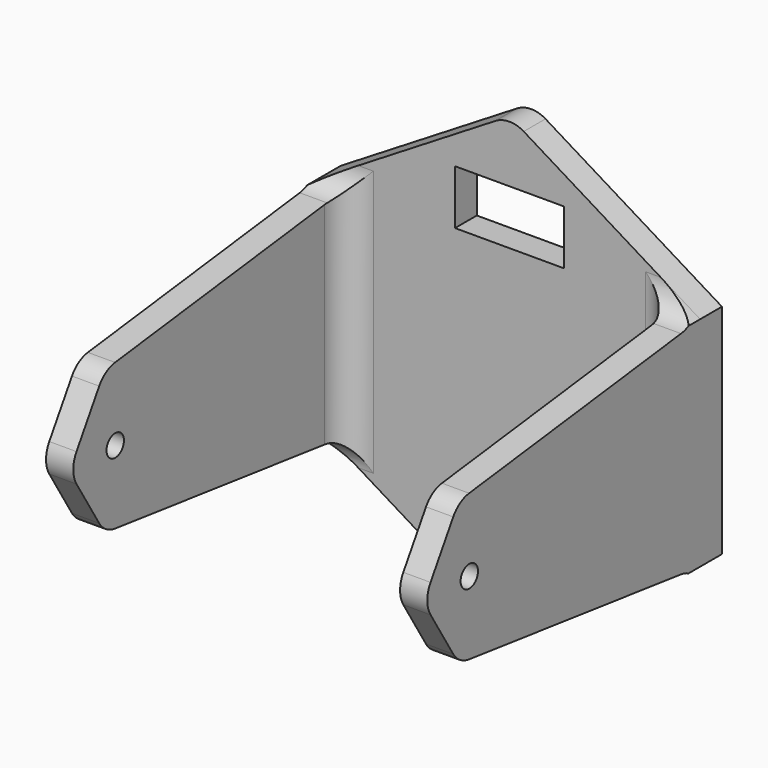
from build123d import *

# Parameters (mm, degrees)
F0_W         = 5
F0_H         = 40
F1_DEPTH     = 70
F3_DEPTH     = 5
F4_R         = 2
F5_DEPTH     = 97.2
F7_DEPTH     = 83.6
F8_T4_DEPTH  = 65
F8_T10_DEPTH = 65
F8_T16_DEPTH = 5
F8_T21_DEPTH = 5
F8_T26_DEPTH = 5
F8_T31_DEPTH = 5
F8_T37_DEPTH = 16.0458347789
F8_T42_DEPTH = 65
F8_T50_DEPTH = 16.0458347789
F8_T55_DEPTH = 65
F8_T63_DEPTH = 16.0458347789
F8_T68_DEPTH = 65
F8_T76_DEPTH = 65
F8_T81_DEPTH = 16.0458347789
F8_T85_DEPTH = 20.294112478
F9_W         = 20
F9_H         = 10
F10_DEPTH    = 25


# Not quite as in the source:
# - a fillet or chamfer that OpenCascade refuses, or shapes differently, is made with other operations: its cross-section is extruded or revolved along the edge and cut away or added


with BuildPart() as f1:
    # F0 (on Front) → F1 (new body)
    with BuildSketch(Plane.XZ):
        with Locations((-32.5, 0)):
            Rectangle(F0_W, F0_H)
    extrude(amount=F1_DEPTH)



with BuildPart() as f1b:
    # F0 (on Front) → F1, piece 2 (new body)
    with BuildSketch(Plane.XZ):
        with Locations((32.5, 0)):
            Rectangle(F0_W, F0_H)
    extrude(amount=F1_DEPTH)


with BuildPart() as f1_1:
    add(f1.part)

    add(f1b.part)  # F3 merges F1b
    # F2 (on face) → F3 (join)
    with BuildSketch(Plane(origin=(0, 0, 0), x_dir=(-1, 0, 0), z_dir=(0, 1, 0))):
        Polygon((-35, -20), (0, -41.4117574692), (35, -20), (35, 20), (0, 41.4117574692), (-35, 20), align=None)
    extrude(amount=F3_DEPTH)

    # F4 (on face) → F5 (cut)
    with BuildSketch(Plane(origin=(-35, 0, 0), x_dir=(0, -1, 0), z_dir=(-1, 0, 0))):
        with Locations((52.9787652194, 0)):
            Circle(F4_R)
    extrude(amount=-F5_DEPTH, mode=Mode.SUBTRACT)

    # F6 (on face) → F7 (cut)
    with BuildSketch(Plane(origin=(-35, 0, 0), x_dir=(0, -1, 0), z_dir=(-1, 0, 0))):
        with BuildLine():
            Line((98.4306931496, 40.8057309687), (0, 20))
            Line((0, 20), (53.01884554, 13.4261534673))
            ThreePointArc((53.01884554, 13.4261534673), (55.107028482, 12.6702755654), (56.6618948527, 11.084636902))
            Line((56.6618948527, 11.084636902), (61.8706015463, 2.6204867239))
            ThreePointArc((61.8706015463, 2.6204867239), (62.6123097139, 0), (61.8706015463, -2.6204867239))
            Line((61.8706015463, -2.6204867239), (56.6618948527, -11.084636902))
            ThreePointArc((56.6618948527, -11.084636902), (55.107028482, -12.6702755654), (53.01884554, -13.4261534673))
            Line((53.01884554, -13.4261534673), (0, -20))
            Line((0, -20), (98.4306931496, -42.0177839696))
            Line((98.4306931496, -42.0177839696), (98.4306931496, 40.8057309687))
        make_face()
    extrude(amount=-F7_DEPTH, mode=Mode.SUBTRACT)

    # F8: fillet of radius 5 on 8 edges, made by hand


with BuildPart() as f8_tool2:
    # F8_s3 → F8_t4 (new body)
    with BuildSketch(Plane.XY.offset(32.5)):
        with BuildLine():
            ThreePointArc((25, 0), (28.5355339059, -1.4644660941), (30, -5))
            Line((30, -5), (30, 0))
            Line((30, 0), (25, 0))
        make_face()
    extrude(amount=-F8_T4_DEPTH)

    split(bisect_by=Plane(origin=(0, -2.4422683248, 19.6971813136), x_dir=(1, 0, 0), z_dir=(0, 0.1230485039, -0.9924006578)), keep=Keep.TOP)

    split(bisect_by=Plane(origin=(0, -2.4422683248, -19.6971813136), x_dir=(1, 0, 0), z_dir=(0, 0.1230485039, 0.9924006578)), keep=Keep.TOP)


with BuildPart() as f1_2:
    add(f1_1.part)

    # F8_t1: union F8_tool2
    add(f8_tool2.part)


with BuildPart() as f8_tool8:
    # F8_s9 → F8_t10 (new body)
    with BuildSketch(Plane.XY.offset(-32.5)):
        with BuildLine():
            ThreePointArc((-25, 0), (-28.5355339059, -1.4644660941), (-30, -5))
            Line((-30, -5), (-30, 0))
            Line((-30, 0), (-25, 0))
        make_face()
    extrude(amount=F8_T10_DEPTH)

    split(bisect_by=Plane(origin=(0, -2.4422683248, -19.6971813136), x_dir=(1, 0, 0), z_dir=(0, 0.1230485039, 0.9924006578)), keep=Keep.TOP)

    split(bisect_by=Plane(origin=(0, -2.4422683248, 19.6971813136), x_dir=(1, 0, 0), z_dir=(0, 0.1230485039, -0.9924006578)), keep=Keep.TOP)


with BuildPart() as f1_3:
    add(f1_2.part)

    # F8_t7: union F8_tool8
    add(f8_tool8.part)


with BuildPart() as f8_tool14:
    # F8_s15 → F8_t16 (new body)
    with BuildSketch(Plane.YZ.offset(35)):
        with BuildLine():
            ThreePointArc((-4.3847574804, 19.4563306223), (-1.2532539052, 21.1074588458), (0, 24.4183339115))
            Line((0, 24.4183339115), (0, 20))
            Line((0, 20), (-4.3847574804, 19.4563306223))
        make_face()
    extrude(amount=-F8_T16_DEPTH)

    split(bisect_by=Plane(origin=(18.4348816442, 0, 30.1339513338), x_dir=(0, 1, 0), z_dir=(-0.5218557601, 0, -0.8530337424)), keep=Keep.TOP)


with BuildPart() as f1_4:
    add(f1_3.part)

    # F8_t13: union F8_tool14
    add(f8_tool14.part)


with BuildPart() as f8_tool19:
    # F8_s20 → F8_t21 (new body)
    with BuildSketch(Plane.YZ.offset(-30)):
        with BuildLine():
            ThreePointArc((0, 24.4183339115), (-1.2532539052, 21.1074588458), (-4.3847574804, 19.4563306223))
            Line((-4.3847574804, 19.4563306223), (0, 20))
            Line((0, 20), (0, 24.4183339115))
        make_face()
    extrude(amount=-F8_T21_DEPTH)

    split(bisect_by=Plane(origin=(-18.4348816442, 0, 30.1339513338), x_dir=(0, 1, 0), z_dir=(0.5218557601, 0, -0.8530337424)), keep=Keep.TOP)


with BuildPart() as f1_5:
    add(f1_4.part)

    # F8_t18: union F8_tool19
    add(f8_tool19.part)


with BuildPart() as f8_tool24:
    # F8_s25 → F8_t26 (new body)
    with BuildSketch(Plane.YZ.offset(-35)):
        with BuildLine():
            ThreePointArc((0, -24.4183339115), (-1.2532539052, -21.1074588458), (-4.3847574804, -19.4563306223))
            Line((-4.3847574804, -19.4563306223), (0, -20))
            Line((0, -20), (0, -24.4183339115))
        make_face()
    extrude(amount=F8_T26_DEPTH)

    split(bisect_by=Plane(origin=(-18.4348816442, 0, -30.1339513338), x_dir=(0, 1, 0), z_dir=(0.5218557601, 0, 0.8530337424)), keep=Keep.TOP)


with BuildPart() as f1_6:
    add(f1_5.part)

    # F8_t23: union F8_tool24
    add(f8_tool24.part)


with BuildPart() as f8_tool29:
    # F8_s30 → F8_t31 (new body)
    with BuildSketch(Plane.YZ.offset(30)):
        with BuildLine():
            ThreePointArc((-4.3847574804, -19.4563306223), (-1.2532539052, -21.1074588458), (0, -24.4183339115))
            Line((0, -24.4183339115), (0, -20))
            Line((0, -20), (-4.3847574804, -19.4563306223))
        make_face()
    extrude(amount=F8_T31_DEPTH)

    split(bisect_by=Plane(origin=(18.4348816442, 0, -30.1339513338), x_dir=(0, 1, 0), z_dir=(-0.5218557601, 0, 0.8530337424)), keep=Keep.TOP)


with BuildPart() as f1_7:
    add(f1_6.part)

    # F8_t28: union F8_tool29
    add(f8_tool29.part)


with BuildPart() as f8_tool35:
    # F8_s36 → F8_t37 (new body)
    with BuildSketch(Plane.YZ.offset(35)):
        with BuildLine():
            ThreePointArc((-4.3847574804, 19.4563306223), (-1.2532539052, 21.1074588458), (0, 24.4183339115))
            Line((0, 24.4183339115), (0, 20))
            Line((0, 20), (-4.3847574804, 19.4563306223))
        make_face()
    extrude(amount=-F8_T37_DEPTH)

    split(bisect_by=Plane(origin=(18.4348816442, 0, 30.1339513338), x_dir=(0, 1, 0), z_dir=(-0.5218557601, 0, -0.8530337424)), keep=Keep.TOP)

    split(bisect_by=Plane.YZ.offset(30), keep=Keep.BOTTOM)


with BuildPart() as f8_tool40:
    # F8_s41 → F8_t42 (new body)
    with BuildSketch(Plane.XY.offset(32.5)):
        with BuildLine():
            ThreePointArc((25, 0), (28.5355339059, -1.4644660941), (30, -5))
            Line((30, -5), (30, 0))
            Line((30, 0), (25, 0))
        make_face()
    extrude(amount=-F8_T42_DEPTH)

    split(bisect_by=Plane(origin=(18.4348816442, 0, 30.1339513338), x_dir=(0, 1, 0), z_dir=(-0.5218557601, 0, -0.8530337424)), keep=Keep.TOP)

    split(bisect_by=Plane(origin=(0, -2.4422683248, 19.6971813136), x_dir=(1, 0, 0), z_dir=(0, -0.1230485039, 0.9924006578)), keep=Keep.TOP)


with BuildPart() as f8_tool35_1:
    add(f8_tool35.part)

    # F8_t45: intersect F8_tool40
    add(f8_tool40.part, mode=Mode.INTERSECT)


with BuildPart() as f1_8:
    add(f1_7.part)

    # F8_t33: union F8_tool35
    add(f8_tool35_1.part)


with BuildPart() as f8_tool48:
    # F8_s49 → F8_t50 (new body)
    with BuildSketch(Plane.YZ.offset(18.9541652211)):
        with BuildLine():
            ThreePointArc((-4.3847574804, -19.4563306223), (-1.2532539052, -21.1074588458), (0, -24.4183339115))
            Line((0, -24.4183339115), (0, -20))
            Line((0, -20), (-4.3847574804, -19.4563306223))
        make_face()
    extrude(amount=F8_T50_DEPTH)

    split(bisect_by=Plane(origin=(18.4348816442, 0, -30.1339513338), x_dir=(0, 1, 0), z_dir=(-0.5218557601, 0, 0.8530337424)), keep=Keep.TOP)

    split(bisect_by=Plane.YZ.offset(30), keep=Keep.BOTTOM)


with BuildPart() as f8_tool53:
    # F8_s54 → F8_t55 (new body)
    with BuildSketch(Plane.XY.offset(32.5)):
        with BuildLine():
            ThreePointArc((25, 0), (28.5355339059, -1.4644660941), (30, -5))
            Line((30, -5), (30, 0))
            Line((30, 0), (25, 0))
        make_face()
    extrude(amount=-F8_T55_DEPTH)

    split(bisect_by=Plane(origin=(18.4348816442, 0, -30.1339513338), x_dir=(0, 1, 0), z_dir=(-0.5218557601, 0, 0.8530337424)), keep=Keep.TOP)

    split(bisect_by=Plane(origin=(0, -2.4422683248, -19.6971813136), x_dir=(1, 0, 0), z_dir=(0, -0.1230485039, -0.9924006578)), keep=Keep.TOP)


with BuildPart() as f8_tool48_1:
    add(f8_tool48.part)

    # F8_t58: intersect F8_tool53
    add(f8_tool53.part, mode=Mode.INTERSECT)


with BuildPart() as f1_9:
    add(f1_8.part)

    # F8_t46: union F8_tool48
    add(f8_tool48_1.part)


with BuildPart() as f8_tool61:
    # F8_s62 → F8_t63 (new body)
    with BuildSketch(Plane.YZ.offset(-35)):
        with BuildLine():
            ThreePointArc((0, -24.4183339115), (-1.2532539052, -21.1074588458), (-4.3847574804, -19.4563306223))
            Line((-4.3847574804, -19.4563306223), (0, -20))
            Line((0, -20), (0, -24.4183339115))
        make_face()
    extrude(amount=F8_T63_DEPTH)

    split(bisect_by=Plane(origin=(-18.4348816442, 0, -30.1339513338), x_dir=(0, 1, 0), z_dir=(0.5218557601, 0, 0.8530337424)), keep=Keep.TOP)

    split(bisect_by=Plane.YZ.offset(-30), keep=Keep.TOP)


with BuildPart() as f8_tool66:
    # F8_s67 → F8_t68 (new body)
    with BuildSketch(Plane.XY.offset(-32.5)):
        with BuildLine():
            ThreePointArc((-25, 0), (-28.5355339059, -1.4644660941), (-30, -5))
            Line((-30, -5), (-30, 0))
            Line((-30, 0), (-25, 0))
        make_face()
    extrude(amount=F8_T68_DEPTH)

    split(bisect_by=Plane(origin=(-18.4348816442, 0, -30.1339513338), x_dir=(0, 1, 0), z_dir=(0.5218557601, 0, 0.8530337424)), keep=Keep.TOP)

    split(bisect_by=Plane(origin=(0, -2.4422683248, -19.6971813136), x_dir=(1, 0, 0), z_dir=(0, -0.1230485039, -0.9924006578)), keep=Keep.TOP)


with BuildPart() as f8_tool61_1:
    add(f8_tool61.part)

    # F8_t71: intersect F8_tool66
    add(f8_tool66.part, mode=Mode.INTERSECT)


with BuildPart() as f1_10:
    add(f1_9.part)

    # F8_t59: union F8_tool61
    add(f8_tool61_1.part)


with BuildPart() as f8_tool74:
    # F8_s75 → F8_t76 (new body)
    with BuildSketch(Plane.XY.offset(-32.5)):
        with BuildLine():
            ThreePointArc((-25, 0), (-28.5355339059, -1.4644660941), (-30, -5))
            Line((-30, -5), (-30, 0))
            Line((-30, 0), (-25, 0))
        make_face()
    extrude(amount=F8_T76_DEPTH)

    split(bisect_by=Plane(origin=(-18.4348816442, 0, 30.1339513338), x_dir=(0, 1, 0), z_dir=(0.5218557601, 0, -0.8530337424)), keep=Keep.TOP)

    split(bisect_by=Plane(origin=(0, -2.4422683248, 19.6971813136), x_dir=(1, 0, 0), z_dir=(0, -0.1230485039, 0.9924006578)), keep=Keep.TOP)


with BuildPart() as f8_tool79:
    # F8_s80 → F8_t81 (new body)
    with BuildSketch(Plane.YZ.offset(-18.9541652211)):
        with BuildLine():
            ThreePointArc((0, 24.4183339115), (-1.2532539052, 21.1074588458), (-4.3847574804, 19.4563306223))
            Line((-4.3847574804, 19.4563306223), (0, 20))
            Line((0, 20), (0, 24.4183339115))
        make_face()
    extrude(amount=-F8_T81_DEPTH)

    split(bisect_by=Plane(origin=(-18.4348816442, 0, 30.1339513338), x_dir=(0, 1, 0), z_dir=(0.5218557601, 0, -0.8530337424)), keep=Keep.TOP)

    split(bisect_by=Plane.YZ.offset(-30), keep=Keep.TOP)


with BuildPart() as f8_tool74_1:
    add(f8_tool74.part)

    # F8_t84: intersect F8_tool79
    add(f8_tool79.part, mode=Mode.INTERSECT)


with BuildPart() as f1_11:
    add(f1_10.part)

    # F8_t72: union F8_tool74
    add(f8_tool74_1.part)

    # F8_s86 → F8_t85 (cut)
    with BuildSketch(Plane.XZ.offset(-12.647056239)):
        with BuildLine():
            ThreePointArc((-2.6092788007, 39.8154933306), (0, 40.5503246188), (2.6092788007, 39.8154933306))
            Line((2.6092788007, 39.8154933306), (0, 41.4117574692))
            Line((0, 41.4117574692), (-2.6092788007, 39.8154933306))
        make_face()
        with BuildLine():
            ThreePointArc((-2.6092788007, -39.8154933306), (0, -40.5503246188), (2.6092788007, -39.8154933306))
            Line((2.6092788007, -39.8154933306), (0, -41.4117574692))
            Line((0, -41.4117574692), (-2.6092788007, -39.8154933306))
        make_face()
    extrude(amount=F8_T85_DEPTH, mode=Mode.SUBTRACT)

    # F9 (on face) → F10 (cut)
    with BuildSketch(Plane.XZ):
        with Locations((0, 25.0998503715)):
            Rectangle(F9_W, F9_H)
    extrude(amount=-F10_DEPTH, mode=Mode.SUBTRACT)


solid = f1_11.part
